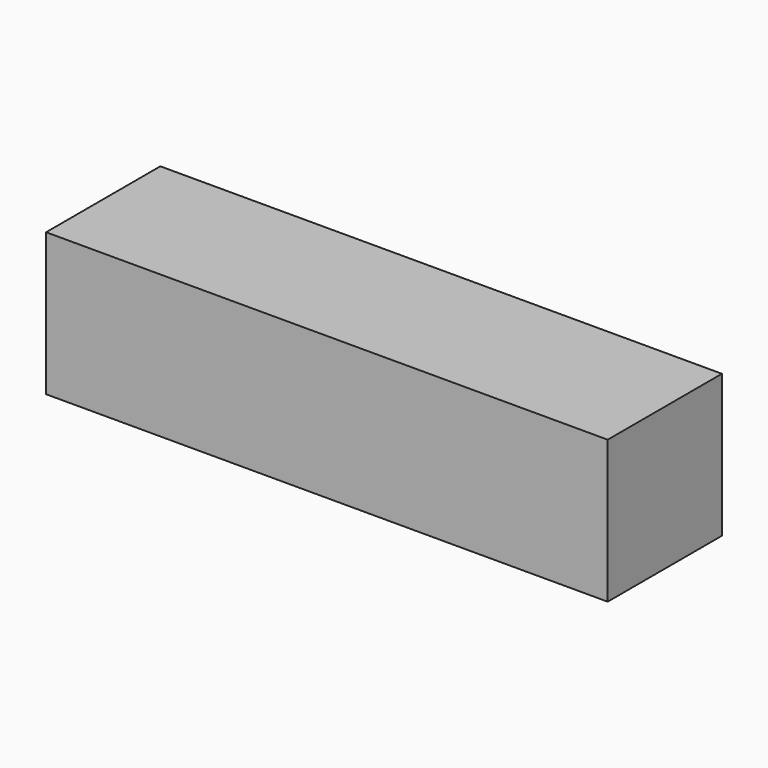
from build123d import *

# Parameters (mm, degrees)
F1_DEPTH = 6


with BuildPart() as f1:
    # F0 (on Front) → F1 (new body)
    with BuildSketch(Plane.XZ):
        Polygon((-34.4077316761, 43.5570870492), (-58.0077316761, 43.5570870492), (-58.0077316761, 37.5632319629), (-52.0077316761, 37.5632319629), (-34.4077316761, 37.5632319629), align=None)
    extrude(amount=F1_DEPTH)


solid = f1.part
